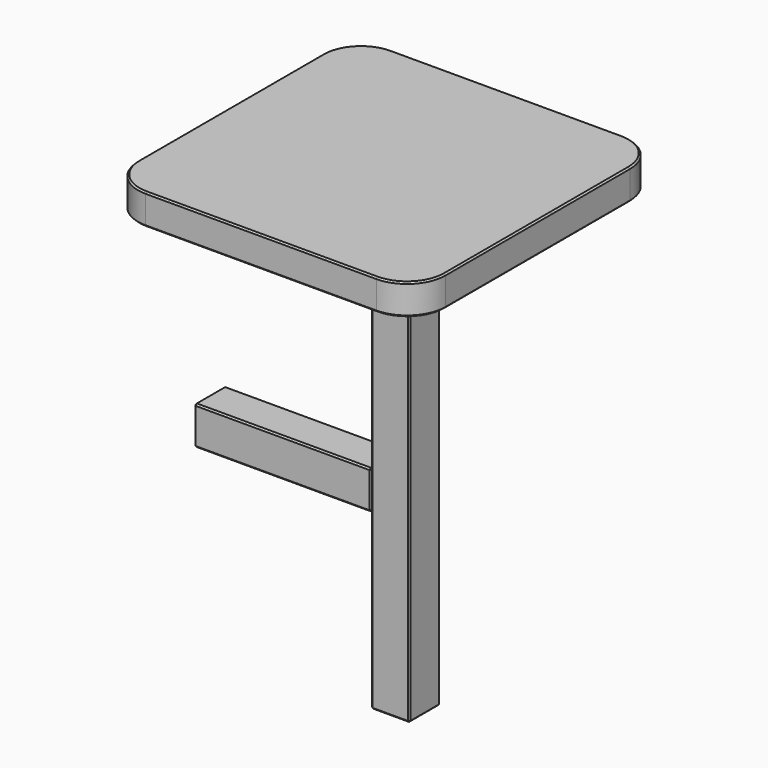
from build123d import *

# Parameters (mm, degrees)
F0_W      = 400
F0_H      = 400
F1_DEPTH  = 40
F2_W      = 50
F2_H      = 50
F3_DEPTH  = 20
F4_R      = 50
F5_DEPTH  = 500
F6_W      = 50
F6_H      = 50
F7_DEPTH  = 230
F8_SIZE   = 2
F8_2_SIZE = 2
F8_3_SIZE = 2


with BuildPart() as f1:
    # F0 (on Top) → F1 (new body)
    with BuildSketch(Plane.XY):
        Rectangle(F0_W, F0_H)
    extrude(amount=F1_DEPTH)

    # F2 (on face) → F3 (cut)
    with BuildSketch(Plane(origin=(0, 0, 0), x_dir=(1, 0, 0), z_dir=(0, 0, -1))):
        with Locations((140, 140)):
            Rectangle(F2_W, F2_H)
        with Locations((140, -140)):
            Rectangle(F2_W, F2_H)
        with Locations((-140, -140)):
            Rectangle(F2_W, F2_H)
        with Locations((-140, 140)):
            Rectangle(F2_W, F2_H)
    extrude(amount=-F3_DEPTH, mode=Mode.SUBTRACT)

    # F4
    f4_edges = [f1.edges().sort_by_distance(p)[0] for p in [
        (200, -200, 20),
        (200, 200, 20),
        (-200, 200, 20),
        (-200, -200, 20),
    ]]
    fillet(f4_edges, radius=F4_R)


with BuildPart() as f5:
    # F5 (new): a face of the model
    f5_faces = [f1.part.faces().sort_by_distance(p)[0] for p in [
        (140, -140, 20),
    ]]
    extrude(f5_faces, amount=F5_DEPTH)

    # F8#2
    f8_2_edges = [f5.edges().sort_by_distance(p)[0] for p in [
        (140, -115, 20),
        (165, -140, 20),
        (140, -165, 20),
        (115, -140, 20),
        (115, -165, -230),
        (115, -115, -230),
        (115, -140, -480),
        (165, -165, -230),
        (140, -165, -480),
        (140, -115, -480),
        (165, -115, -230),
        (165, -140, -480),
    ]]
    chamfer(f8_2_edges, length=F8_2_SIZE)


with BuildPart() as f7:
    # F6 (on face) → F7 (new body, through all)
    with BuildSketch(Plane(origin=(115, 0, 0), x_dir=(0, -1, 0), z_dir=(-1, 0, 0))):
        with Locations((140, -230)):
            Rectangle(F6_W, F6_H)
    extrude(amount=F7_DEPTH)

    # F8#3
    f8_3_edges = [f7.edges().sort_by_distance(p)[0] for p in [
        (115, -165, -230),
        (115, -115, -230),
        (0, -165, -205),
        (0, -115, -205),
        (115, -140, -205),
        (0, -165, -255),
        (115, -140, -255),
        (0, -115, -255),
        (-115, -165, -230),
        (-115, -140, -205),
        (-115, -115, -230),
        (-115, -140, -255),
    ]]
    chamfer(f8_3_edges, length=F8_3_SIZE)


with BuildPart() as f1_1:
    add(f1.part)

    # F8
    f8_edges = [f1_1.edges().sort_by_distance(p)[0] for p in [
        (-185.355339, -185.355339, 0),
        (185.355339, -185.355339, 40),
        (-185.355339, 185.355339, 40),
        (-185.355339, 185.355339, 0),
        (0, -200, 0),
        (0, -200, 40),
        (-200, 0, 0),
        (0, 200, 40),
        (-185.355339, -185.355339, 40),
        (-200, 0, 40),
        (200, 0, 40),
        (185.355339, 185.355339, 40),
        (150, -200, 20),
        (150, 200, 20),
        (185.355339, 185.355339, 0),
        (-200, -150, 20),
        (-140, -165, 0),
        (200, 150, 20),
        (140, 165, 20),
        (200, -150, 20),
        (-200, 150, 20),
        (200, 0, 0),
        (115, -140, 0),
        (0, 200, 0),
        (-150, 200, 20),
        (-140, 115, 20),
        (140, -115, 20),
        (-150, -200, 20),
        (185.355339, -185.355339, 0),
        (140, 115, 0),
        (-115, -140, 0),
        (140, 165, 0),
        (165, -140, 20),
        (-115, 140, 20),
        (165, 140, 0),
        (-140, 165, 0),
        (165, 165, 10),
        (140, -165, 20),
        (-165, -140, 20),
        (-165, -140, 0),
        (-165, 140, 0),
        (-140, 165, 20),
        (-165, 140, 20),
        (140, 115, 20),
        (-115, 140, 0),
        (-140, -165, 20),
        (-165, -165, 10),
        (115, -140, 20),
        (115, 115, 10),
        (-165, 115, 10),
        (-165, -115, 10),
        (165, 140, 20),
        (-115, -165, 10),
        (140, -165, 0),
        (-165, 165, 10),
        (-140, -115, 0),
        (115, 140, 20),
        (165, -140, 0),
        (-115, -115, 10),
        (115, 140, 0),
        (-115, 115, 10),
        (-140, 115, 0),
        (115, 165, 10),
        (-115, -140, 20),
        (-140, -115, 20),
        (140, -115, 0),
        (165, 115, 10),
        (-115, 165, 10),
        (165, -165, 10),
        (165, -115, 10),
        (115, -115, 10),
        (115, -165, 10),
    ]]
    chamfer(f8_edges, length=F8_SIZE)


solid = Compound([f5.part, f7.part, f1_1.part])
